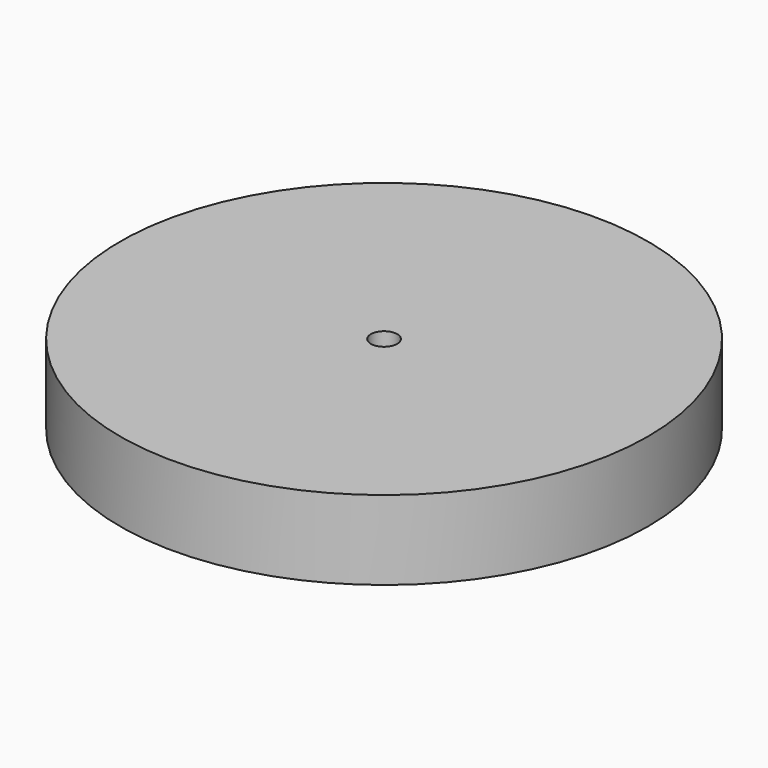
from build123d import *


# Not quite as in the source:
# - ends of sketch curves that miss each other by under 0.0002 mm in the source are joined


with BuildPart() as f1:
    # F0 (on Front) → F1 (revolve)
    with BuildSketch(Plane.XZ):
        Polygon((10, 149.9999946356), (10, 135), (4.1, 135), (4.1, 125), (20.5, 125), (20.5, 90), (200, 90), (200, 150), align=None)
    revolve(axis=Axis((0, 0, 50), (0, 0, 1)))


solid = f1.part
